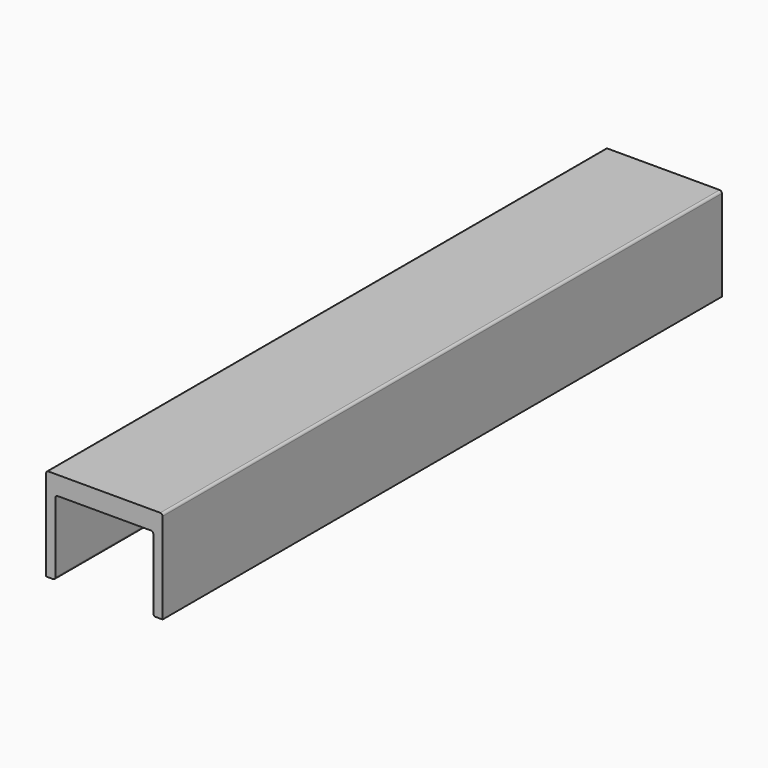
from build123d import *

# Parameters (mm, degrees)
F1_DEPTH = 75
F3_R     = 0.5


with BuildPart() as f1:
    # F0 (on Front) → F1 (new body, symmetric)
    with BuildSketch(Plane.XZ):
        Polygon((25, 20), (0, 20), (0, 0), (2, 0), (2, 16), (23, 16), (23, 0), (25, 0), align=None)
    extrude(amount=F1_DEPTH, both=True)

    # F3
    f3_edges = [f1.edges().sort_by_distance(p)[0] for p in [
        (0, 0, 20),
        (25, 0, 20),
        (23, 0, 0),
        (23, 0, 16),
        (2, 0, 16),
        (2, 0, 0),
    ]]
    fillet(f3_edges, radius=F3_R)


solid = f1.part
